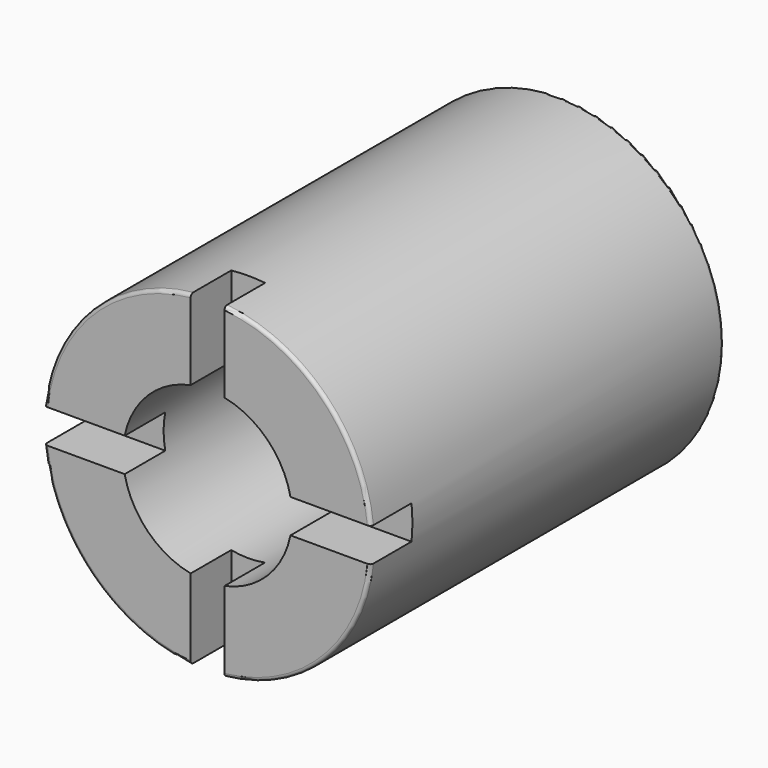
from build123d import *

# Parameters (mm, degrees)
F0_R     = 12.319
F1_DEPTH = 33.02
F3_R     = 6.35
F4_DEPTH = 25.4
F5_R     = 0.254
F7_DEPTH = 3.81


with BuildPart() as f1:
    # F0 (on Front) → F1 (new body)
    with BuildSketch(Plane.XZ):
        Circle(F0_R)
    extrude(amount=F1_DEPTH)

    # F3 (on face) → F4 (cut)
    with BuildSketch(Plane.XZ.offset(33.02)):
        Circle(F3_R)
    extrude(amount=-F4_DEPTH, mode=Mode.SUBTRACT)

    # F5
    f5_edges = [f1.edges().sort_by_distance(p)[0] for p in [
        (-12.319, -33.02, 0),
        (-12.319, 0, 0),
    ]]
    fillet(f5_edges, radius=F5_R)

    # F6 (on face) → F7 (cut)
    with BuildSketch(Plane.XZ.offset(33.02)):
        with BuildLine():
            ThreePointArc((-1.27, 6.2217039467), (0, 6.35), (1.27, 6.2217039467))
            Line((1.27, 6.2217039467), (1.27, 12.2533612123))
            ThreePointArc((1.27, 12.2533612123), (0, 12.319), (-1.27, 12.2533612123))
            Line((-1.27, 12.2533612123), (-1.27, 6.2217039467))
        make_face()
        with BuildLine():
            Line((-6.2217039467, 1.27), (-12.2533612123, 1.27))
            ThreePointArc((-12.2533612123, 1.27), (-12.319, 0), (-12.2533612123, -1.27))
            Line((-12.2533612123, -1.27), (-6.2217039467, -1.27))
            ThreePointArc((-6.2217039467, -1.27), (-6.35, 0), (-6.2217039467, 1.27))
        make_face()
        with BuildLine():
            Line((-1.27, -6.2217039467), (-1.27, -12.2533612123))
            ThreePointArc((-1.27, -12.2533612123), (0, -12.319), (1.27, -12.2533612123))
            Line((1.27, -12.2533612123), (1.27, -6.2217039467))
            ThreePointArc((1.27, -6.2217039467), (0, -6.35), (-1.27, -6.2217039467))
        make_face()
        with BuildLine():
            Line((6.2217039467, -1.27), (12.2533612123, -1.27))
            ThreePointArc((12.2533612123, -1.27), (12.319, 0), (12.2533612123, 1.27))
            Line((12.2533612123, 1.27), (6.2217039467, 1.27))
            ThreePointArc((6.2217039467, 1.27), (6.35, 0), (6.2217039467, -1.27))
        make_face()
    extrude(amount=-F7_DEPTH, mode=Mode.SUBTRACT)


solid = f1.part
